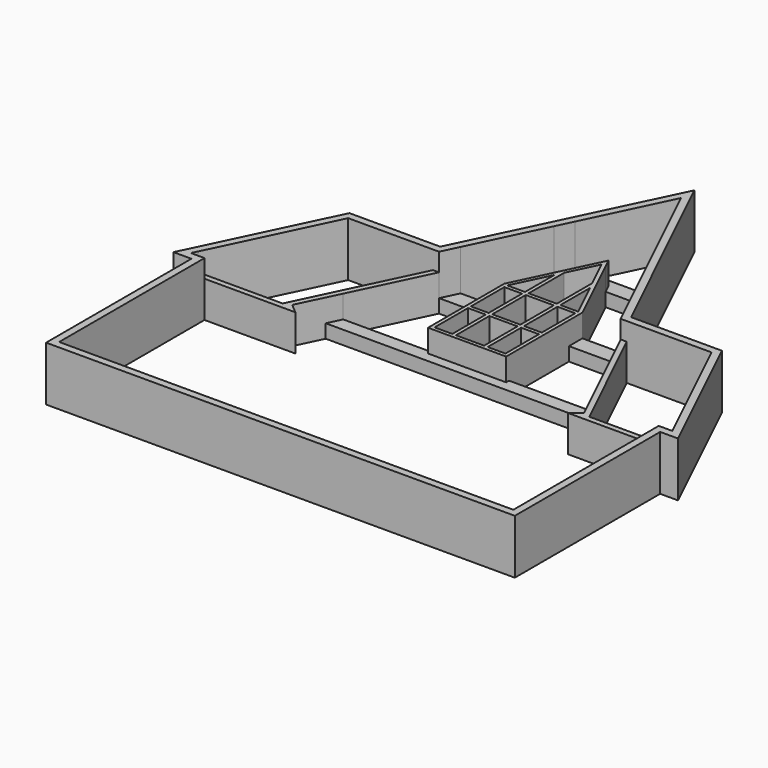
from build123d import *

# Parameters (mm, degrees)
F1_DEPTH = 15.24
F2_DEPTH = 10.16
F0_W     = 4.953
F0_H     = 11.6882068259
F0_W_2   = 7.8621185967
F3_DEPTH = 10.16
F4_DEPTH = 3.81


# Not quite as in the source:
# - a feature names something its author has since deleted; it is built from what else it names


with BuildPart() as f1:
    # F0 (on Top) → F1 (new body)
    with BuildSketch(Plane.XY):
        Polygon((56.8358146836, 36.3690045497), (31.4358146836, 36.3690045497), (4.7581588602, 91.852396227), (-21.9194969632, 36.3690045497), (-23.4601999485, 36.3690045497), (-47.3194969632, 36.3690045497), (-63.1618590029, 3.4205332163), (-65.7835588108, -2.0319997298), (-60.7738408696, -2.0319997298), (-60.7738408696, -52.8319997298), (70.29015859, -52.8319997298), (70.29015859, -2.0319997298), (75.2998765312, -2.0319997298), (72.6781767233, 3.4205332163), align=None)
        Polygon((68.2581588602, -50.8), (-58.7418411398, -50.8), (-58.7418411398, 0), (-62.5518411398, 0), (-61.8190678495, 1.524), (-46.0418411398, 34.3370048199), (-22.332856425, 34.3370048199), (-20.6418411398, 34.3370048199), (-18.376729311, 39.0479167388), (-8.5820728345, 59.4185506966), (-6.3910428531, 63.9753894023), (4.7581588602, 87.1631660812), (15.9073605735, 63.9753894023), (18.0983905549, 59.4185506966), (27.8930470314, 39.0479167388), (30.1581588602, 34.3370048199), (31.8491741455, 34.3370048199), (55.5581588602, 34.3370048199), (71.3353855699, 1.524), (72.0681588602, 0), (68.2581588602, 0), align=None, mode=Mode.SUBTRACT)
    extrude(amount=F1_DEPTH)

    # F0 (on Top) → F2 (join)
    with BuildSketch(Plane.XY):
        Polygon((-62.5518411398, 0), (-58.7418411398, 0), (-33.3418411398, 0), (-36.0511744731, 2.2891336547), (-32.5333754715, 9.6053469359), (-30.7009610057, 13.4163478047), (-20.6418411398, 34.3370048199), (-22.332856425, 34.3370048199), (-38.1100831348, 1.524), (-58.7418411398, 1.524), (-61.8190678495, 1.524), align=None)
        Polygon((42.8581588602, 0), (68.2581588602, 0), (72.0681588602, 0), (71.3353855699, 1.524), (68.2581588602, 1.524), (47.6264008552, 1.524), (31.8491741455, 34.3370048199), (30.1581588602, 34.3370048199), (40.2172787262, 13.4163478047), (42.0496931919, 9.6053469359), (45.5674921935, 2.2891336547), align=None)
    extrude(amount=F2_DEPTH)



with BuildPart() as f3:
    # F0 (on Top) → F3 (new body)
    with BuildSketch(Plane.XY):
        Polygon((-6.1638411398, 34.3370048199), (-6.1638411398, 13.4163478047), (-5.1478411398, 13.4163478047), (-5.1478411398, 25.1078879876), (-0.1948411398, 25.1078879876), (-0.1948411398, 13.4163478047), (0.8297724999, 13.4163478047), (0.8297724999, 25.1078879876), (8.6918910965, 25.1078879876), (8.6918910965, 13.4163478047), (9.7111588602, 13.4163478047), (9.7111588602, 25.1078879876), (14.6641588602, 25.1078879876), (14.6641588602, 13.4163478047), (15.6801588602, 13.4163478047), (15.6801588602, 34.3370048199), (15.6801588602, 39.0479167388), (5.8855023837, 59.4185506966), (4.7581588602, 59.4185506966), (3.6308153367, 59.4185506966), (-6.1638411398, 39.0479167388), align=None)
        with Locations((-2.6713411398, 31.9604512176)):
            Rectangle(F0_W, F0_H, mode=Mode.SUBTRACT)
        Polygon((-5.1478411398, 38.8163478047), (-0.1948411398, 49.1174492506), (-0.1948411398, 38.8163478047), align=None, mode=Mode.SUBTRACT)
        with Locations((4.7608317982, 31.9604512176)):
            Rectangle(F0_W_2, F0_H, mode=Mode.SUBTRACT)
        with Locations((12.1876588602, 31.9604512176)):
            Rectangle(F0_W, F0_H, mode=Mode.SUBTRACT)
        Polygon((9.7111588602, 49.1174492506), (14.6641588602, 38.8163478047), (9.7111588602, 38.8163478047), align=None, mode=Mode.SUBTRACT)
        Polygon((0.8297724999, 51.2484100915), (4.7581588602, 59.4185506966), (8.6918910965, 51.2372918984), (8.6918910965, 38.8163478047), (0.8297724999, 38.8163478047), align=None, mode=Mode.SUBTRACT)
        Polygon((4.7581588602, 61.7631660812), (3.6308153367, 59.4185506966), (4.7581588602, 59.4185506966), (5.8855023837, 59.4185506966), align=None)
        Polygon((-5.1478411398, 13.4163478047), (-6.1638411398, 13.4163478047), (-6.1638411398, 12.4003478047), (15.6801588602, 12.4003478047), (15.6801588602, 13.4163478047), (14.6641588602, 13.4163478047), (9.7111588602, 13.4163478047), (8.6918910965, 13.4163478047), (0.8297724999, 13.4163478047), (-0.1948411398, 13.4163478047), align=None)
    extrude(amount=F3_DEPTH)


with BuildPart() as f1_1:
    add(f1.part)

    add(f3.part)  # F4 merges F3
    # F0 (on Top) → F4 (join)
    with BuildSketch(Plane.XY):
        Polygon((-30.7009610057, 13.4163478047), (-32.5333754715, 9.6053469359), (42.0496931919, 9.6053469359), (40.2172787262, 13.4163478047), (15.6801588602, 13.4163478047), (15.6801588602, 12.4003478047), (-6.1638411398, 12.4003478047), (-6.1638411398, 13.4163478047), align=None)
        Polygon((-18.376729311, 39.0479167388), (-20.6418411398, 34.3370048199), (-6.1638411398, 34.3370048199), (-6.1638411398, 39.0479167388), align=None)
        Polygon((15.6801588602, 34.3370048199), (30.1581588602, 34.3370048199), (27.8930470314, 39.0479167388), (15.6801588602, 39.0479167388), align=None)
        Polygon((-6.3910428531, 63.9753894023), (-8.5820728345, 59.4185506966), (3.6308153367, 59.4185506966), (4.7581588602, 61.7631660812), (5.8855023837, 59.4185506966), (18.0983905549, 59.4185506966), (15.9073605735, 63.9753894023), align=None)
    extrude(amount=F4_DEPTH)


solid = f1_1.part
